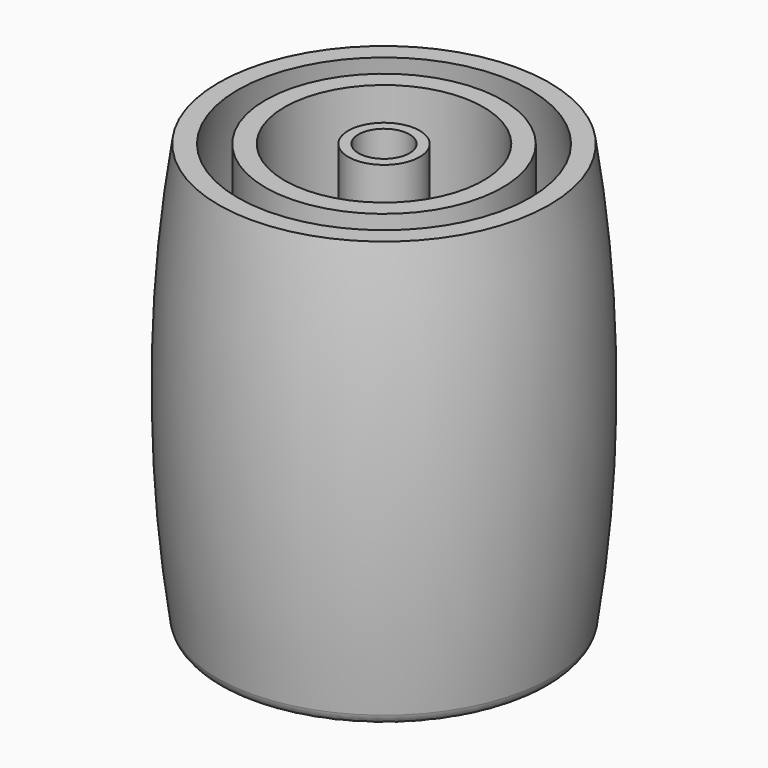
from build123d import *

# Parameters (mm, degrees)
F2_R = 2


# Not quite as in the source:
# - two fillets or chamfers of one size are made in one step
# - a feature names something its author has since deleted; it is built from what else it names


with BuildPart() as f1:
    # F0 (on Front) → F1 (revolve)
    with BuildSketch(Plane.XZ):
        with BuildLine():
            Line((-25.9578547239, 0), (-4, 0))
            Line((-4, 0), (-4, 67))
            Line((-4, 67), (-5.6, 67))
            Line((-5.6, 67), (-5.6, 3))
            Line((-5.6, 3), (-15.6, 3))
            Line((-15.6, 3), (-15.6, 67))
            Line((-15.6, 67), (-18.6, 67))
            Line((-18.6, 67), (-18.6, 3))
            Line((-18.6, 3), (-23.3657418773, 3))
            ThreePointArc((-23.3657418773, 3), (-25.4947508744, 35.0162748691), (-22.9226189658, 67))
            Line((-22.9226189658, 67), (-25.9578547239, 67))
            ThreePointArc((-25.9578547239, 67), (-28.5, 33.5), (-25.9578547239, 0))
        make_face()
    revolve(axis=Axis((0, 0, 33.5), (0, 0, 1)))

    # F2
    f2_edges = [f1.edges().sort_by_distance(p)[0] for p in [
        (15.6, 0, 3),
        (23.365742, 0, 3),
        (18.6, 0, 3),
        (4, 0, 0),
        (25.957855, 0, 0),
        (5.6, 0, 3),
    ]]
    fillet(f2_edges, radius=F2_R)


solid = f1.part
